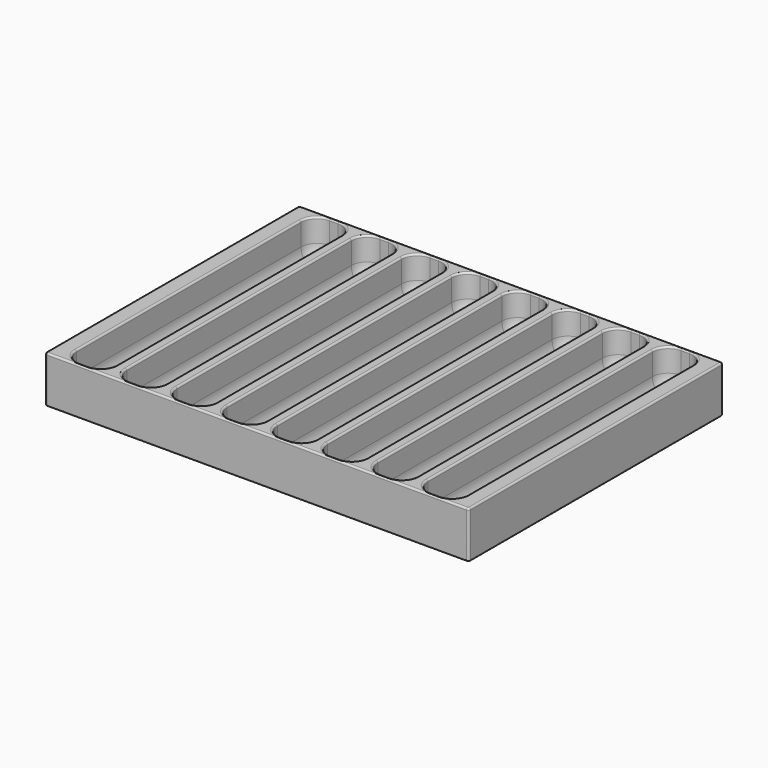
from build123d import *

# Parameters (mm, degrees)
F0_W          = 190
F0_H          = 142.5
F1_DEPTH      = 21
F2_W          = 18
F2_H          = 16
F3_DEPTH      = 70
F12_R         = 7.1
F13_T1_DEPTH  = 125.8
F13_T3_DEPTH  = 146.5
F13_T5_DEPTH  = 194
F13_T7_DEPTH  = 3.8
F13_T9_DEPTH  = 3.8
F13_T11_DEPTH = 3.8
F13_T13_DEPTH = 3.8
F13_T15_DEPTH = 3.8
F13_T17_DEPTH = 3.8
F13_T19_DEPTH = 3.8
F13_T21_DEPTH = 3.8
F13_T24_ANGLE = 90
F13_T26_ANGLE = 90
F13_T28_ANGLE = 90
F13_T30_ANGLE = 90
F13_T32_ANGLE = 90
F13_T34_ANGLE = 90
F13_T36_ANGLE = 90
F13_T38_ANGLE = 90
F13_T40_ANGLE = 90
F13_T42_ANGLE = 90
F13_T44_ANGLE = 90
F13_T46_ANGLE = 90
F13_T48_ANGLE = 90
F13_T50_ANGLE = 90
F13_T52_ANGLE = 90
F13_T54_ANGLE = 90
F13_T56_ANGLE = 90
F13_T58_ANGLE = 90
F13_T60_ANGLE = 90
F13_T62_ANGLE = 90
F13_T64_ANGLE = 90
F13_T66_ANGLE = 90
F13_T68_ANGLE = 90
F13_T70_ANGLE = 90
F13_T72_ANGLE = 90
F13_T74_ANGLE = 90
F13_T76_ANGLE = 90
F13_T78_ANGLE = 90
F13_T80_ANGLE = 90
F13_T82_ANGLE = 90
F13_T84_ANGLE = 90
F13_T86_ANGLE = 90
F14_T1_DEPTH  = 23.5000000002
F14_T4_ANGLE  = 90
F14_T6_ANGLE  = 90
F14_T8_ANGLE  = 90
F14_T10_ANGLE = 90
F15_R         = 0.5


# Not quite as in the source:
# - a fillet or chamfer that OpenCascade refuses, or shapes differently, is made with other operations: its cross-section is extruded or revolved along the edge and cut away or added


with BuildPart() as f1:
    # F0 (on Top) → F1 (new body)
    with BuildSketch(Plane.XY):
        Rectangle(F0_W, F0_H)
    extrude(amount=F1_DEPTH)


with BuildPart() as f3:
    # F2 (on Front) → F3 (new body, symmetric)
    with BuildSketch(Plane.XZ):
        with Locations((-78.4749761224, 18.5186266899)):
            Rectangle(F2_W, F2_H)
        with BuildLine():
            ThreePointArc((-87.4749761224, 10.5186266899), (-78.4749761224, 1.5186266899), (-69.4749761224, 10.5186266899))
            Line((-69.4749761224, 10.5186266899), (-87.4749761224, 10.5186266899))
        make_face()
    extrude(amount=F3_DEPTH, both=True)


with BuildPart() as f4_1:
    # F4: copy of F3
    add(f3.part.moved(Location((22.5, 0, 0))))


with BuildPart() as f5_1:
    # F5: copy of F4_1
    add(f4_1.part.moved(Location((22.5, 0, 0))))


with BuildPart() as f6_1:
    # F6: copy of F5_1
    add(f5_1.part.moved(Location((22.5, 0, 0))))


with BuildPart() as f7_1:
    # F7: copy of F6_1
    add(f6_1.part.moved(Location((22.5, 0, 0))))


with BuildPart() as f8_1:
    # F8: copy of F7_1
    add(f7_1.part.moved(Location((22.5, 0, 0))))


with BuildPart() as f9_1:
    # F9: copy of F8_1
    add(f8_1.part.moved(Location((22.5, 0, 0))))


with BuildPart() as f10_1:
    # F10: copy of F9_1
    add(f9_1.part.moved(Location((22.5, 0, 0))))


with BuildPart() as f1_1:
    add(f1.part)

    # F11: cut F3, F4_1, F5_1, F6_1, F7_1, F8_1, F9_1, F10_1
    add(f3.part, mode=Mode.SUBTRACT)
    add(f4_1.part, mode=Mode.SUBTRACT)
    add(f5_1.part, mode=Mode.SUBTRACT)
    add(f6_1.part, mode=Mode.SUBTRACT)
    add(f7_1.part, mode=Mode.SUBTRACT)
    add(f8_1.part, mode=Mode.SUBTRACT)
    add(f9_1.part, mode=Mode.SUBTRACT)
    add(f10_1.part, mode=Mode.SUBTRACT)

    # F12
    f12_edges = [f1_1.edges().sort_by_distance(p)[0] for p in [
        (-78.474976, 70, 1.518627),
        (-55.974976, 70, 1.518627),
        (-33.474976, 70, 1.518627),
        (-10.974976, 70, 1.518627),
        (34.025024, 70, 1.518627),
        (11.525024, 70, 1.518627),
        (56.525024, 70, 1.518627),
        (79.025024, 70, 1.518627),
        (79.025024, -70, 1.518627),
        (56.525024, -70, 1.518627),
        (34.025024, -70, 1.518627),
        (11.525024, -70, 1.518627),
        (-10.974976, -70, 1.518627),
        (-33.474976, -70, 1.518627),
        (-55.974976, -70, 1.518627),
        (-78.474976, -70, 1.518627),
    ]]
    fillet(f12_edges, radius=F12_R)

    # F13: fillet of radius 0.8 on 12 edges, made by hand

    # F13_s2 → F13_t1 (cut)
    with BuildSketch(Plane.XZ.offset(-62.9)):
        with BuildLine():
            ThreePointArc((-88.2749761224, 21), (-87.7092906974, 20.7656854249), (-87.4749761224, 20.2))
            Line((-87.4749761224, 20.2), (-87.4749761224, 21))
            Line((-87.4749761224, 21), (-88.2749761224, 21))
        make_face()
        with BuildLine():
            ThreePointArc((-65.7749761224, 21), (-65.2092906974, 20.7656854249), (-64.9749761224, 20.2))
            Line((-64.9749761224, 20.2), (-64.9749761224, 21))
            Line((-64.9749761224, 21), (-65.7749761224, 21))
        make_face()
        with BuildLine():
            ThreePointArc((-43.2749761224, 21), (-42.7092906974, 20.7656854249), (-42.4749761224, 20.2))
            Line((-42.4749761224, 20.2), (-42.4749761224, 21))
            Line((-42.4749761224, 21), (-43.2749761224, 21))
        make_face()
        with BuildLine():
            ThreePointArc((-20.7749761224, 21), (-20.2092906974, 20.7656854249), (-19.9749761224, 20.2))
            Line((-19.9749761224, 20.2), (-19.9749761224, 21))
            Line((-19.9749761224, 21), (-20.7749761224, 21))
        make_face()
        with BuildLine():
            ThreePointArc((1.7250238776, 21), (2.2907093026, 20.7656854249), (2.5250238776, 20.2))
            Line((2.5250238776, 20.2), (2.5250238776, 21))
            Line((2.5250238776, 21), (1.7250238776, 21))
        make_face()
        with BuildLine():
            ThreePointArc((24.2250238776, 21), (24.7907093026, 20.7656854249), (25.0250238776, 20.2))
            Line((25.0250238776, 20.2), (25.0250238776, 21))
            Line((25.0250238776, 21), (24.2250238776, 21))
        make_face()
        with BuildLine():
            ThreePointArc((46.7250238776, 21), (47.2907093026, 20.7656854249), (47.5250238776, 20.2))
            Line((47.5250238776, 20.2), (47.5250238776, 21))
            Line((47.5250238776, 21), (46.7250238776, 21))
        make_face()
        with BuildLine():
            ThreePointArc((69.2250238776, 21), (69.7907093026, 20.7656854249), (70.0250238776, 20.2))
            Line((70.0250238776, 20.2), (70.0250238776, 21))
            Line((70.0250238776, 21), (69.2250238776, 21))
        make_face()
        with BuildLine():
            ThreePointArc((88.8250238776, 21), (88.2593384527, 20.7656854249), (88.0250238776, 20.2))
            Line((88.0250238776, 20.2), (88.0250238776, 21))
            Line((88.0250238776, 21), (88.8250238776, 21))
        make_face()
        with BuildLine():
            ThreePointArc((66.3250238776, 21), (65.7593384527, 20.7656854249), (65.5250238776, 20.2))
            Line((65.5250238776, 20.2), (65.5250238776, 21))
            Line((65.5250238776, 21), (66.3250238776, 21))
        make_face()
        with BuildLine():
            ThreePointArc((43.8250238776, 21), (43.2593384527, 20.7656854249), (43.0250238776, 20.2))
            Line((43.0250238776, 20.2), (43.0250238776, 21))
            Line((43.0250238776, 21), (43.8250238776, 21))
        make_face()
        with BuildLine():
            ThreePointArc((21.3250238776, 21), (20.7593384527, 20.7656854249), (20.5250238776, 20.2))
            Line((20.5250238776, 20.2), (20.5250238776, 21))
            Line((20.5250238776, 21), (21.3250238776, 21))
        make_face()
        with BuildLine():
            ThreePointArc((-1.1749761224, 21), (-1.7406615473, 20.7656854249), (-1.9749761224, 20.2))
            Line((-1.9749761224, 20.2), (-1.9749761224, 21))
            Line((-1.9749761224, 21), (-1.1749761224, 21))
        make_face()
        with BuildLine():
            ThreePointArc((-23.6749761224, 21), (-24.2406615473, 20.7656854249), (-24.4749761224, 20.2))
            Line((-24.4749761224, 20.2), (-24.4749761224, 21))
            Line((-24.4749761224, 21), (-23.6749761224, 21))
        make_face()
        with BuildLine():
            ThreePointArc((-46.1749761224, 21), (-46.7406615473, 20.7656854249), (-46.9749761224, 20.2))
            Line((-46.9749761224, 20.2), (-46.9749761224, 21))
            Line((-46.9749761224, 21), (-46.1749761224, 21))
        make_face()
        with BuildLine():
            ThreePointArc((-68.6749761224, 21), (-69.2406615473, 20.7656854249), (-69.4749761224, 20.2))
            Line((-69.4749761224, 20.2), (-69.4749761224, 21))
            Line((-69.4749761224, 21), (-68.6749761224, 21))
        make_face()
    extrude(amount=F13_T1_DEPTH, mode=Mode.SUBTRACT)

    # F13_s4 → F13_t3 (cut)
    with BuildSketch(Plane.XZ.offset(-73.25)):
        with BuildLine():
            ThreePointArc((-94.2, 21), (-94.7656854249, 20.7656854249), (-95, 20.2))
            Line((-95, 20.2), (-95, 21))
            Line((-95, 21), (-94.2, 21))
        make_face()
        with BuildLine():
            ThreePointArc((94.2, 21), (94.7656854249, 20.7656854249), (95, 20.2))
            Line((95, 20.2), (95, 21))
            Line((95, 21), (94.2, 21))
        make_face()
    extrude(amount=F13_T3_DEPTH, mode=Mode.SUBTRACT)

    # F13_s6 → F13_t5 (cut)
    with BuildSketch(Plane.YZ.offset(-97)):
        with BuildLine():
            ThreePointArc((-70.45, 21), (-71.0156854249, 20.7656854249), (-71.25, 20.2))
            Line((-71.25, 20.2), (-71.25, 21))
            Line((-71.25, 21), (-70.45, 21))
        make_face()
        with BuildLine():
            ThreePointArc((70.45, 21), (71.0156854249, 20.7656854249), (71.25, 20.2))
            Line((71.25, 20.2), (71.25, 21))
            Line((71.25, 21), (70.45, 21))
        make_face()
    extrude(amount=F13_T5_DEPTH, mode=Mode.SUBTRACT)

    # F13_s8 → F13_t7 (cut)
    with BuildSketch(Plane.YZ.offset(77.1250238776)):
        with BuildLine():
            ThreePointArc((-70.8, 21), (-70.2343145751, 20.7656854249), (-70, 20.2))
            Line((-70, 20.2), (-70, 21))
            Line((-70, 21), (-70.8, 21))
        make_face()
        with BuildLine():
            ThreePointArc((70.8, 21), (70.2343145751, 20.7656854249), (70, 20.2))
            Line((70, 20.2), (70, 21))
            Line((70, 21), (70.8, 21))
        make_face()
    extrude(amount=F13_T7_DEPTH, mode=Mode.SUBTRACT)

    # F13_s10 → F13_t9 (cut)
    with BuildSketch(Plane.YZ.offset(54.6250238776)):
        with BuildLine():
            ThreePointArc((-70.8, 21), (-70.2343145751, 20.7656854249), (-70, 20.2))
            Line((-70, 20.2), (-70, 21))
            Line((-70, 21), (-70.8, 21))
        make_face()
        with BuildLine():
            ThreePointArc((70.8, 21), (70.2343145751, 20.7656854249), (70, 20.2))
            Line((70, 20.2), (70, 21))
            Line((70, 21), (70.8, 21))
        make_face()
    extrude(amount=F13_T9_DEPTH, mode=Mode.SUBTRACT)

    # F13_s12 → F13_t11 (cut)
    with BuildSketch(Plane.YZ.offset(32.1250238776)):
        with BuildLine():
            ThreePointArc((-70.8, 21), (-70.2343145751, 20.7656854249), (-70, 20.2))
            Line((-70, 20.2), (-70, 21))
            Line((-70, 21), (-70.8, 21))
        make_face()
        with BuildLine():
            ThreePointArc((70.8, 21), (70.2343145751, 20.7656854249), (70, 20.2))
            Line((70, 20.2), (70, 21))
            Line((70, 21), (70.8, 21))
        make_face()
    extrude(amount=F13_T11_DEPTH, mode=Mode.SUBTRACT)

    # F13_s14 → F13_t13 (cut)
    with BuildSketch(Plane.YZ.offset(9.6250238776)):
        with BuildLine():
            ThreePointArc((-70.8, 21), (-70.2343145751, 20.7656854249), (-70, 20.2))
            Line((-70, 20.2), (-70, 21))
            Line((-70, 21), (-70.8, 21))
        make_face()
        with BuildLine():
            ThreePointArc((70.8, 21), (70.2343145751, 20.7656854249), (70, 20.2))
            Line((70, 20.2), (70, 21))
            Line((70, 21), (70.8, 21))
        make_face()
    extrude(amount=F13_T13_DEPTH, mode=Mode.SUBTRACT)

    # F13_s16 → F13_t15 (cut)
    with BuildSketch(Plane.YZ.offset(-12.8749761224)):
        with BuildLine():
            ThreePointArc((-70.8, 21), (-70.2343145751, 20.7656854249), (-70, 20.2))
            Line((-70, 20.2), (-70, 21))
            Line((-70, 21), (-70.8, 21))
        make_face()
        with BuildLine():
            ThreePointArc((70.8, 21), (70.2343145751, 20.7656854249), (70, 20.2))
            Line((70, 20.2), (70, 21))
            Line((70, 21), (70.8, 21))
        make_face()
    extrude(amount=F13_T15_DEPTH, mode=Mode.SUBTRACT)

    # F13_s18 → F13_t17 (cut)
    with BuildSketch(Plane.YZ.offset(-35.3749761224)):
        with BuildLine():
            ThreePointArc((-70.8, 21), (-70.2343145751, 20.7656854249), (-70, 20.2))
            Line((-70, 20.2), (-70, 21))
            Line((-70, 21), (-70.8, 21))
        make_face()
        with BuildLine():
            ThreePointArc((70.8, 21), (70.2343145751, 20.7656854249), (70, 20.2))
            Line((70, 20.2), (70, 21))
            Line((70, 21), (70.8, 21))
        make_face()
    extrude(amount=F13_T17_DEPTH, mode=Mode.SUBTRACT)

    # F13_s20 → F13_t19 (cut)
    with BuildSketch(Plane.YZ.offset(-57.8749761224)):
        with BuildLine():
            ThreePointArc((-70.8, 21), (-70.2343145751, 20.7656854249), (-70, 20.2))
            Line((-70, 20.2), (-70, 21))
            Line((-70, 21), (-70.8, 21))
        make_face()
        with BuildLine():
            ThreePointArc((70.8, 21), (70.2343145751, 20.7656854249), (70, 20.2))
            Line((70, 20.2), (70, 21))
            Line((70, 21), (70.8, 21))
        make_face()
    extrude(amount=F13_T19_DEPTH, mode=Mode.SUBTRACT)

    # F13_s22 → F13_t21 (cut)
    with BuildSketch(Plane.YZ.offset(-80.3749761224)):
        with BuildLine():
            ThreePointArc((-70.8, 21), (-70.2343145751, 20.7656854249), (-70, 20.2))
            Line((-70, 20.2), (-70, 21))
            Line((-70, 21), (-70.8, 21))
        make_face()
        with BuildLine():
            ThreePointArc((70.8, 21), (70.2343145751, 20.7656854249), (70, 20.2))
            Line((70, 20.2), (70, 21))
            Line((70, 21), (70.8, 21))
        make_face()
    extrude(amount=F13_T21_DEPTH, mode=Mode.SUBTRACT)

    # F13_s23 → F13_t24 (revolve, cut)
    with BuildSketch(Plane.YZ.offset(77.1250238776)):
        with BuildLine():
            ThreePointArc((70.8, 21), (70.2343145751, 20.7656854249), (70, 20.2))
            Line((70, 20.2), (70, 21))
            Line((70, 21), (70.8, 21))
        make_face()
    revolve(axis=Axis((77.1250238776, 62.9, 21), (0, 0, 1)), revolution_arc=F13_T24_ANGLE, mode=Mode.SUBTRACT)

    # F13_s25 → F13_t26 (revolve, cut)
    with BuildSketch(Plane.YZ.offset(77.1250238776)):
        with BuildLine():
            ThreePointArc((-70.8, 21), (-70.2343145751, 20.7656854249), (-70, 20.2))
            Line((-70, 20.2), (-70, 21))
            Line((-70, 21), (-70.8, 21))
        make_face()
    revolve(axis=Axis((77.1250238776, -62.9, 21), (0, 0, -1)), revolution_arc=F13_T26_ANGLE, mode=Mode.SUBTRACT)

    # F13_s27 → F13_t28 (revolve, cut)
    with BuildSketch(Plane.YZ.offset(80.9250238776)):
        with BuildLine():
            ThreePointArc((-70.8, 21), (-70.2343145751, 20.7656854249), (-70, 20.2))
            Line((-70, 20.2), (-70, 21))
            Line((-70, 21), (-70.8, 21))
        make_face()
    revolve(axis=Axis((80.9250238776, -62.9, 21), (0, 0, 1)), revolution_arc=F13_T28_ANGLE, mode=Mode.SUBTRACT)

    # F13_s29 → F13_t30 (revolve, cut)
    with BuildSketch(Plane.YZ.offset(80.9250238776)):
        with BuildLine():
            ThreePointArc((70.8, 21), (70.2343145751, 20.7656854249), (70, 20.2))
            Line((70, 20.2), (70, 21))
            Line((70, 21), (70.8, 21))
        make_face()
    revolve(axis=Axis((80.9250238776, 62.9, 21), (0, 0, -1)), revolution_arc=F13_T30_ANGLE, mode=Mode.SUBTRACT)

    # F13_s31 → F13_t32 (revolve, cut)
    with BuildSketch(Plane.YZ.offset(54.6250238776)):
        with BuildLine():
            ThreePointArc((70.8, 21), (70.2343145751, 20.7656854249), (70, 20.2))
            Line((70, 20.2), (70, 21))
            Line((70, 21), (70.8, 21))
        make_face()
    revolve(axis=Axis((54.6250238776, 62.9, 21), (0, 0, 1)), revolution_arc=F13_T32_ANGLE, mode=Mode.SUBTRACT)

    # F13_s33 → F13_t34 (revolve, cut)
    with BuildSketch(Plane.YZ.offset(54.6250238776)):
        with BuildLine():
            ThreePointArc((-70.8, 21), (-70.2343145751, 20.7656854249), (-70, 20.2))
            Line((-70, 20.2), (-70, 21))
            Line((-70, 21), (-70.8, 21))
        make_face()
    revolve(axis=Axis((54.6250238776, -62.9, 21), (0, 0, -1)), revolution_arc=F13_T34_ANGLE, mode=Mode.SUBTRACT)

    # F13_s35 → F13_t36 (revolve, cut)
    with BuildSketch(Plane.YZ.offset(58.4250238776)):
        with BuildLine():
            ThreePointArc((-70.8, 21), (-70.2343145751, 20.7656854249), (-70, 20.2))
            Line((-70, 20.2), (-70, 21))
            Line((-70, 21), (-70.8, 21))
        make_face()
    revolve(axis=Axis((58.4250238776, -62.9, 21), (0, 0, 1)), revolution_arc=F13_T36_ANGLE, mode=Mode.SUBTRACT)

    # F13_s37 → F13_t38 (revolve, cut)
    with BuildSketch(Plane.YZ.offset(58.4250238776)):
        with BuildLine():
            ThreePointArc((70.8, 21), (70.2343145751, 20.7656854249), (70, 20.2))
            Line((70, 20.2), (70, 21))
            Line((70, 21), (70.8, 21))
        make_face()
    revolve(axis=Axis((58.4250238776, 62.9, 21), (0, 0, -1)), revolution_arc=F13_T38_ANGLE, mode=Mode.SUBTRACT)

    # F13_s39 → F13_t40 (revolve, cut)
    with BuildSketch(Plane.YZ.offset(32.1250238776)):
        with BuildLine():
            ThreePointArc((70.8, 21), (70.2343145751, 20.7656854249), (70, 20.2))
            Line((70, 20.2), (70, 21))
            Line((70, 21), (70.8, 21))
        make_face()
    revolve(axis=Axis((32.1250238776, 62.9, 21), (0, 0, 1)), revolution_arc=F13_T40_ANGLE, mode=Mode.SUBTRACT)

    # F13_s41 → F13_t42 (revolve, cut)
    with BuildSketch(Plane.YZ.offset(32.1250238776)):
        with BuildLine():
            ThreePointArc((-70.8, 21), (-70.2343145751, 20.7656854249), (-70, 20.2))
            Line((-70, 20.2), (-70, 21))
            Line((-70, 21), (-70.8, 21))
        make_face()
    revolve(axis=Axis((32.1250238776, -62.9, 21), (0, 0, -1)), revolution_arc=F13_T42_ANGLE, mode=Mode.SUBTRACT)

    # F13_s43 → F13_t44 (revolve, cut)
    with BuildSketch(Plane.YZ.offset(35.9250238776)):
        with BuildLine():
            ThreePointArc((-70.8, 21), (-70.2343145751, 20.7656854249), (-70, 20.2))
            Line((-70, 20.2), (-70, 21))
            Line((-70, 21), (-70.8, 21))
        make_face()
    revolve(axis=Axis((35.9250238776, -62.9, 21), (0, 0, 1)), revolution_arc=F13_T44_ANGLE, mode=Mode.SUBTRACT)

    # F13_s45 → F13_t46 (revolve, cut)
    with BuildSketch(Plane.YZ.offset(35.9250238776)):
        with BuildLine():
            ThreePointArc((70.8, 21), (70.2343145751, 20.7656854249), (70, 20.2))
            Line((70, 20.2), (70, 21))
            Line((70, 21), (70.8, 21))
        make_face()
    revolve(axis=Axis((35.9250238776, 62.9, 21), (0, 0, -1)), revolution_arc=F13_T46_ANGLE, mode=Mode.SUBTRACT)

    # F13_s47 → F13_t48 (revolve, cut)
    with BuildSketch(Plane.YZ.offset(9.6250238776)):
        with BuildLine():
            ThreePointArc((70.8, 21), (70.2343145751, 20.7656854249), (70, 20.2))
            Line((70, 20.2), (70, 21))
            Line((70, 21), (70.8, 21))
        make_face()
    revolve(axis=Axis((9.6250238776, 62.9, 21), (0, 0, 1)), revolution_arc=F13_T48_ANGLE, mode=Mode.SUBTRACT)

    # F13_s49 → F13_t50 (revolve, cut)
    with BuildSketch(Plane.YZ.offset(9.6250238776)):
        with BuildLine():
            ThreePointArc((-70.8, 21), (-70.2343145751, 20.7656854249), (-70, 20.2))
            Line((-70, 20.2), (-70, 21))
            Line((-70, 21), (-70.8, 21))
        make_face()
    revolve(axis=Axis((9.6250238776, -62.9, 21), (0, 0, -1)), revolution_arc=F13_T50_ANGLE, mode=Mode.SUBTRACT)

    # F13_s51 → F13_t52 (revolve, cut)
    with BuildSketch(Plane.YZ.offset(13.4250238776)):
        with BuildLine():
            ThreePointArc((-70.8, 21), (-70.2343145751, 20.7656854249), (-70, 20.2))
            Line((-70, 20.2), (-70, 21))
            Line((-70, 21), (-70.8, 21))
        make_face()
    revolve(axis=Axis((13.4250238776, -62.9, 21), (0, 0, 1)), revolution_arc=F13_T52_ANGLE, mode=Mode.SUBTRACT)

    # F13_s53 → F13_t54 (revolve, cut)
    with BuildSketch(Plane.YZ.offset(13.4250238776)):
        with BuildLine():
            ThreePointArc((70.8, 21), (70.2343145751, 20.7656854249), (70, 20.2))
            Line((70, 20.2), (70, 21))
            Line((70, 21), (70.8, 21))
        make_face()
    revolve(axis=Axis((13.4250238776, 62.9, 21), (0, 0, -1)), revolution_arc=F13_T54_ANGLE, mode=Mode.SUBTRACT)

    # F13_s55 → F13_t56 (revolve, cut)
    with BuildSketch(Plane.YZ.offset(-12.8749761224)):
        with BuildLine():
            ThreePointArc((70.8, 21), (70.2343145751, 20.7656854249), (70, 20.2))
            Line((70, 20.2), (70, 21))
            Line((70, 21), (70.8, 21))
        make_face()
    revolve(axis=Axis((-12.8749761224, 62.9, 21), (0, 0, 1)), revolution_arc=F13_T56_ANGLE, mode=Mode.SUBTRACT)

    # F13_s57 → F13_t58 (revolve, cut)
    with BuildSketch(Plane.YZ.offset(-12.8749761224)):
        with BuildLine():
            ThreePointArc((-70.8, 21), (-70.2343145751, 20.7656854249), (-70, 20.2))
            Line((-70, 20.2), (-70, 21))
            Line((-70, 21), (-70.8, 21))
        make_face()
    revolve(axis=Axis((-12.8749761224, -62.9, 21), (0, 0, -1)), revolution_arc=F13_T58_ANGLE, mode=Mode.SUBTRACT)

    # F13_s59 → F13_t60 (revolve, cut)
    with BuildSketch(Plane.YZ.offset(-9.0749761224)):
        with BuildLine():
            ThreePointArc((-70.8, 21), (-70.2343145751, 20.7656854249), (-70, 20.2))
            Line((-70, 20.2), (-70, 21))
            Line((-70, 21), (-70.8, 21))
        make_face()
    revolve(axis=Axis((-9.0749761224, -62.9, 21), (0, 0, 1)), revolution_arc=F13_T60_ANGLE, mode=Mode.SUBTRACT)

    # F13_s61 → F13_t62 (revolve, cut)
    with BuildSketch(Plane.YZ.offset(-9.0749761224)):
        with BuildLine():
            ThreePointArc((70.8, 21), (70.2343145751, 20.7656854249), (70, 20.2))
            Line((70, 20.2), (70, 21))
            Line((70, 21), (70.8, 21))
        make_face()
    revolve(axis=Axis((-9.0749761224, 62.9, 21), (0, 0, -1)), revolution_arc=F13_T62_ANGLE, mode=Mode.SUBTRACT)

    # F13_s63 → F13_t64 (revolve, cut)
    with BuildSketch(Plane.YZ.offset(-35.3749761224)):
        with BuildLine():
            ThreePointArc((70.8, 21), (70.2343145751, 20.7656854249), (70, 20.2))
            Line((70, 20.2), (70, 21))
            Line((70, 21), (70.8, 21))
        make_face()
    revolve(axis=Axis((-35.3749761224, 62.9, 21), (0, 0, 1)), revolution_arc=F13_T64_ANGLE, mode=Mode.SUBTRACT)

    # F13_s65 → F13_t66 (revolve, cut)
    with BuildSketch(Plane.YZ.offset(-35.3749761224)):
        with BuildLine():
            ThreePointArc((-70.8, 21), (-70.2343145751, 20.7656854249), (-70, 20.2))
            Line((-70, 20.2), (-70, 21))
            Line((-70, 21), (-70.8, 21))
        make_face()
    revolve(axis=Axis((-35.3749761224, -62.9, 21), (0, 0, -1)), revolution_arc=F13_T66_ANGLE, mode=Mode.SUBTRACT)

    # F13_s67 → F13_t68 (revolve, cut)
    with BuildSketch(Plane.YZ.offset(-31.5749761224)):
        with BuildLine():
            ThreePointArc((-70.8, 21), (-70.2343145751, 20.7656854249), (-70, 20.2))
            Line((-70, 20.2), (-70, 21))
            Line((-70, 21), (-70.8, 21))
        make_face()
    revolve(axis=Axis((-31.5749761224, -62.9, 21), (0, 0, 1)), revolution_arc=F13_T68_ANGLE, mode=Mode.SUBTRACT)

    # F13_s69 → F13_t70 (revolve, cut)
    with BuildSketch(Plane.YZ.offset(-31.5749761224)):
        with BuildLine():
            ThreePointArc((70.8, 21), (70.2343145751, 20.7656854249), (70, 20.2))
            Line((70, 20.2), (70, 21))
            Line((70, 21), (70.8, 21))
        make_face()
    revolve(axis=Axis((-31.5749761224, 62.9, 21), (0, 0, -1)), revolution_arc=F13_T70_ANGLE, mode=Mode.SUBTRACT)

    # F13_s71 → F13_t72 (revolve, cut)
    with BuildSketch(Plane.YZ.offset(-57.8749761224)):
        with BuildLine():
            ThreePointArc((70.8, 21), (70.2343145751, 20.7656854249), (70, 20.2))
            Line((70, 20.2), (70, 21))
            Line((70, 21), (70.8, 21))
        make_face()
    revolve(axis=Axis((-57.8749761224, 62.9, 21), (0, 0, 1)), revolution_arc=F13_T72_ANGLE, mode=Mode.SUBTRACT)

    # F13_s73 → F13_t74 (revolve, cut)
    with BuildSketch(Plane.YZ.offset(-57.8749761224)):
        with BuildLine():
            ThreePointArc((-70.8, 21), (-70.2343145751, 20.7656854249), (-70, 20.2))
            Line((-70, 20.2), (-70, 21))
            Line((-70, 21), (-70.8, 21))
        make_face()
    revolve(axis=Axis((-57.8749761224, -62.9, 21), (0, 0, -1)), revolution_arc=F13_T74_ANGLE, mode=Mode.SUBTRACT)

    # F13_s75 → F13_t76 (revolve, cut)
    with BuildSketch(Plane.YZ.offset(-54.0749761224)):
        with BuildLine():
            ThreePointArc((-70.8, 21), (-70.2343145751, 20.7656854249), (-70, 20.2))
            Line((-70, 20.2), (-70, 21))
            Line((-70, 21), (-70.8, 21))
        make_face()
    revolve(axis=Axis((-54.0749761224, -62.9, 21), (0, 0, 1)), revolution_arc=F13_T76_ANGLE, mode=Mode.SUBTRACT)

    # F13_s77 → F13_t78 (revolve, cut)
    with BuildSketch(Plane.YZ.offset(-54.0749761224)):
        with BuildLine():
            ThreePointArc((70.8, 21), (70.2343145751, 20.7656854249), (70, 20.2))
            Line((70, 20.2), (70, 21))
            Line((70, 21), (70.8, 21))
        make_face()
    revolve(axis=Axis((-54.0749761224, 62.9, 21), (0, 0, -1)), revolution_arc=F13_T78_ANGLE, mode=Mode.SUBTRACT)

    # F13_s79 → F13_t80 (revolve, cut)
    with BuildSketch(Plane.YZ.offset(-80.3749761224)):
        with BuildLine():
            ThreePointArc((70.8, 21), (70.2343145751, 20.7656854249), (70, 20.2))
            Line((70, 20.2), (70, 21))
            Line((70, 21), (70.8, 21))
        make_face()
    revolve(axis=Axis((-80.3749761224, 62.9, 21), (0, 0, 1)), revolution_arc=F13_T80_ANGLE, mode=Mode.SUBTRACT)

    # F13_s81 → F13_t82 (revolve, cut)
    with BuildSketch(Plane.YZ.offset(-80.3749761224)):
        with BuildLine():
            ThreePointArc((-70.8, 21), (-70.2343145751, 20.7656854249), (-70, 20.2))
            Line((-70, 20.2), (-70, 21))
            Line((-70, 21), (-70.8, 21))
        make_face()
    revolve(axis=Axis((-80.3749761224, -62.9, 21), (0, 0, -1)), revolution_arc=F13_T82_ANGLE, mode=Mode.SUBTRACT)

    # F13_s83 → F13_t84 (revolve, cut)
    with BuildSketch(Plane.YZ.offset(-76.5749761224)):
        with BuildLine():
            ThreePointArc((-70.8, 21), (-70.2343145751, 20.7656854249), (-70, 20.2))
            Line((-70, 20.2), (-70, 21))
            Line((-70, 21), (-70.8, 21))
        make_face()
    revolve(axis=Axis((-76.5749761224, -62.9, 21), (0, 0, 1)), revolution_arc=F13_T84_ANGLE, mode=Mode.SUBTRACT)

    # F13_s85 → F13_t86 (revolve, cut)
    with BuildSketch(Plane.YZ.offset(-76.5749761224)):
        with BuildLine():
            ThreePointArc((70.8, 21), (70.2343145751, 20.7656854249), (70, 20.2))
            Line((70, 20.2), (70, 21))
            Line((70, 21), (70.8, 21))
        make_face()
    revolve(axis=Axis((-76.5749761224, 62.9, 21), (0, 0, -1)), revolution_arc=F13_T86_ANGLE, mode=Mode.SUBTRACT)

    # F14: fillet of radius 1 on 4 edges, made by hand

    # F14_s2 → F14_t1 (cut)
    with BuildSketch(Plane.XY.offset(-2.5)):
        with BuildLine():
            ThreePointArc((-94, -71.25), (-94.7071067812, -70.9571067812), (-95, -70.25))
            Line((-95, -70.25), (-95, -71.25))
            Line((-95, -71.25), (-94, -71.25))
        make_face()
        with BuildLine():
            ThreePointArc((-94, 71.25), (-94.7071067812, 70.9571067812), (-95, 70.25))
            Line((-95, 70.25), (-95, 71.25))
            Line((-95, 71.25), (-94, 71.25))
        make_face()
        with BuildLine():
            ThreePointArc((94, -71.25), (94.7071067812, -70.9571067812), (95, -70.25))
            Line((95, -70.25), (95, -71.25))
            Line((95, -71.25), (94, -71.25))
        make_face()
        with BuildLine():
            ThreePointArc((94, 71.25), (94.7071067812, 70.9571067812), (95, 70.25))
            Line((95, 70.25), (95, 71.25))
            Line((95, 71.25), (94, 71.25))
        make_face()
    extrude(amount=F14_T1_DEPTH, mode=Mode.SUBTRACT)

    # F14_s3 → F14_t4 (revolve, cut)
    with BuildSketch(Plane.XZ.offset(-70.25)):
        with BuildLine():
            ThreePointArc((94.1999999998, 21), (94.7656854249, 20.7656854249), (95, 20.1999999998))
            Line((95, 20.1999999998), (95, 21))
            Line((95, 21), (94.1999999998, 21))
        make_face()
    revolve(axis=Axis((94, 70.25, 21), (0, 0, 1)), revolution_arc=F14_T4_ANGLE, mode=Mode.SUBTRACT)

    # F14_s5 → F14_t6 (revolve, cut)
    with BuildSketch(Plane.YZ.offset(94)):
        with BuildLine():
            ThreePointArc((-70.4499999998, 21), (-71.0156854249, 20.7656854249), (-71.25, 20.1999999998))
            Line((-71.25, 20.1999999998), (-71.25, 21))
            Line((-71.25, 21), (-70.4499999998, 21))
        make_face()
    revolve(axis=Axis((94, -70.25, 21), (0, 0, 1)), revolution_arc=F14_T6_ANGLE, mode=Mode.SUBTRACT)

    # F14_s7 → F14_t8 (revolve, cut)
    with BuildSketch(Plane.YZ.offset(-94)):
        with BuildLine():
            ThreePointArc((70.4499999998, 21), (71.0156854249, 20.7656854249), (71.25, 20.1999999998))
            Line((71.25, 20.1999999998), (71.25, 21))
            Line((71.25, 21), (70.4499999998, 21))
        make_face()
    revolve(axis=Axis((-94, 70.25, 21), (0, 0, 1)), revolution_arc=F14_T8_ANGLE, mode=Mode.SUBTRACT)

    # F14_s9 → F14_t10 (revolve, cut)
    with BuildSketch(Plane.XZ.offset(70.25)):
        with BuildLine():
            ThreePointArc((-94.1999999998, 21), (-94.7656854249, 20.7656854249), (-95, 20.1999999998))
            Line((-95, 20.1999999998), (-95, 21))
            Line((-95, 21), (-94.1999999998, 21))
        make_face()
    revolve(axis=Axis((-94, -70.25, 21), (0, 0, 1)), revolution_arc=F14_T10_ANGLE, mode=Mode.SUBTRACT)

    # F15
    f15_edges = [f1_1.edges().sort_by_distance(p)[0] for p in [
        (-94.707107, -70.957107, 0),
        (-95, 0, 0),
        (-94.707107, 70.957107, 0),
        (0, 71.25, 0),
        (94.707107, 70.957107, 0),
        (95, 0, 0),
        (94.707107, -70.957107, 0),
        (0, -71.25, 0),
    ]]
    fillet(f15_edges, radius=F15_R)


solid = f1_1.part
